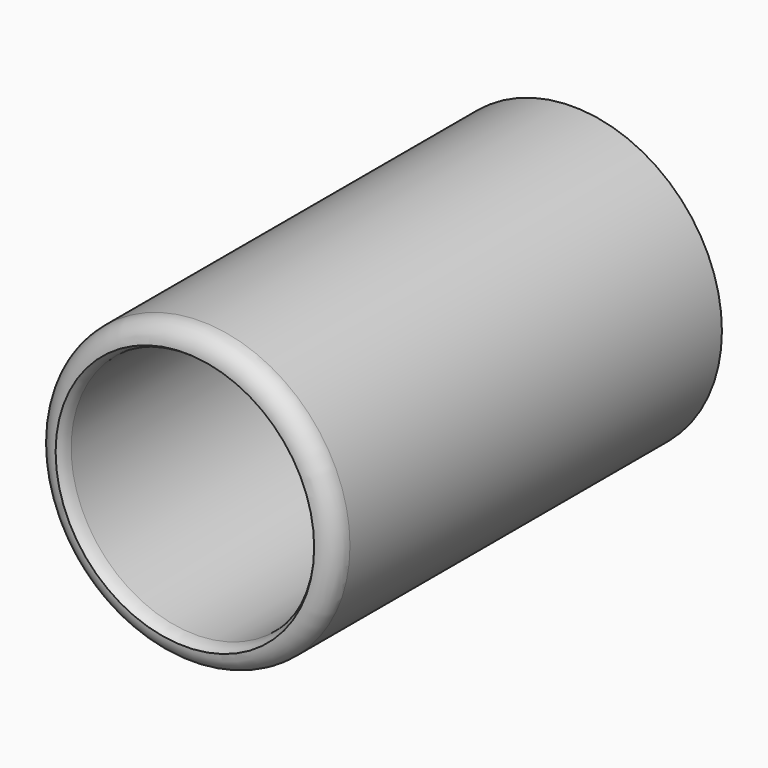
from build123d import *

# Parameters (mm, degrees)
F0_R     = 38.1
F1_DEPTH = 61.9125
F3_T     = -6.35


# Not quite as in the source:
# - a fillet or chamfer that OpenCascade refuses, or shapes differently, is made with other operations: its cross-section is extruded or revolved along the edge and cut away or added
# - a feature of the source that left no trace in its solid (it failed there, or was rolled back) is left out


with BuildPart() as f1:
    # F0 (on Front) → F1 (new body, symmetric)
    with BuildSketch(Plane.XZ):
        Circle(F0_R)
    extrude(amount=F1_DEPTH, both=True)

    # F3
    f3_openings = [f1.faces().sort_by_distance(p)[0] for p in [
        (0, -61.9125, 0),
    ]]
    offset(amount=F3_T, openings=f3_openings)

    # F4: fillet of radius 5.08 on 4 edges, made by hand

    # F4_s1 → F4_t2 (revolve)
    with BuildSketch(Plane.XY):
        with BuildLine():
            ThreePointArc((31.75, 50.4825), (30.2621024484, 54.0746024484), (26.67, 55.5625))
            Line((26.67, 55.5625), (31.75, 55.5625))
            Line((31.75, 55.5625), (31.75, 50.4825))
        make_face()
    revolve(axis=Axis((0, 55.5625, 0), (0, -1, 0)))

    # F4_s3 → F4_t4 (revolve, cut)
    with BuildSketch(Plane.XY):
        with BuildLine():
            ThreePointArc((38.1, -56.8325), (36.6121024484, -60.4246024484), (33.02, -61.9125))
            Line((33.02, -61.9125), (38.1, -61.9125))
            Line((38.1, -61.9125), (38.1, -56.8325))
        make_face()
    revolve(axis=Axis((0, -61.9125, 0), (0, -1, 0)), mode=Mode.SUBTRACT)

    # F4_s5 → F4_t6 (revolve, cut)
    with BuildSketch(Plane.XY):
        with BuildLine():
            ThreePointArc((33.02, -61.9125), (32.0780951188, -60.3484470592), (31.75, -58.5523958349))
            Line((31.75, -58.5523958349), (31.75, -61.9125))
            Line((31.75, -61.9125), (33.02, -61.9125))
        make_face()
    revolve(axis=Axis((0, -61.9125, 0), (0, -1, 0)), mode=Mode.SUBTRACT)


solid = f1.part
